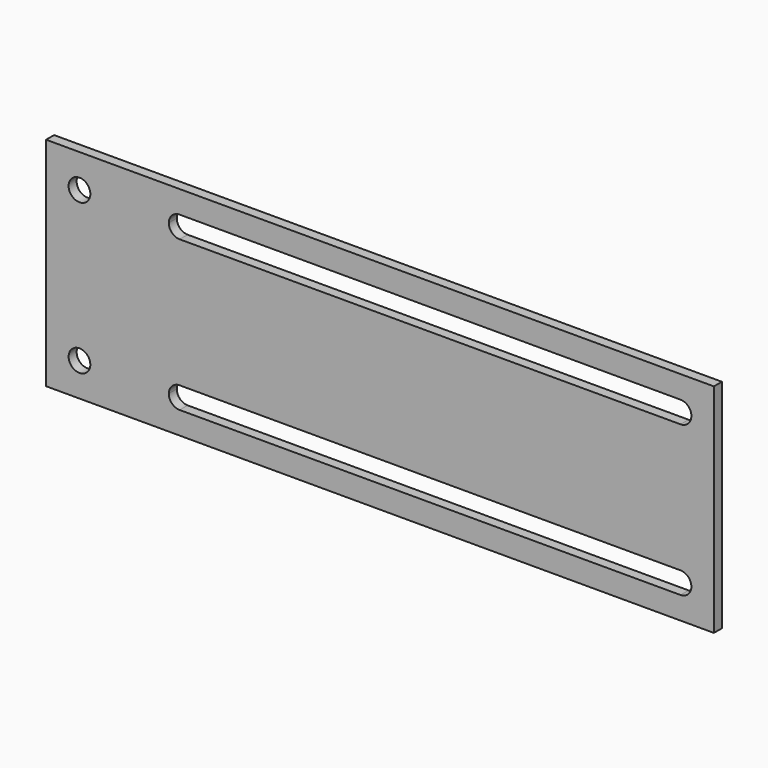
from build123d import *

# Parameters (mm, degrees)
F1_DEPTH = 3


# Not quite as in the source:
# - a feature names something its author has since deleted; it is built from what else it names


with BuildPart() as f1:
    # F0 (on Front) → F1 (new body)
    with BuildSketch(Plane.XZ):
        with BuildLine():
            Line((0, 65), (0, 55))
            Line((0, 55), (6.75, 55))
            ThreePointArc((6.75, 55), (10, 58.25), (13.25, 55))
            Line((13.25, 55), (36.75, 55))
            ThreePointArc((36.75, 55), (37.7019029611, 57.2980970389), (40, 58.25))
            Line((40, 58.25), (100, 58.25))
            Line((100, 58.25), (100, 65))
            Line((100, 65), (0, 65))
        make_face()
        with BuildLine():
            Line((0, 55), (0, 32.5))
            Line((0, 32.5), (30, 32.5))
            Line((30, 32.5), (100, 32.5))
            Line((100, 32.5), (100, 51.75))
            Line((100, 51.75), (40, 51.75))
            ThreePointArc((40, 51.75), (37.7019029611, 52.7019029611), (36.75, 55))
            Line((36.75, 55), (13.25, 55))
            ThreePointArc((13.25, 55), (10, 51.75), (6.75, 55))
            Line((6.75, 55), (0, 55))
        make_face()
        with BuildLine():
            Line((0, 32.5), (0, 10))
            Line((0, 10), (6.75, 10))
            ThreePointArc((6.75, 10), (10, 13.25), (13.25, 10))
            Line((13.25, 10), (30, 10))
            Line((30, 10), (30, 32.5))
            Line((30, 32.5), (0, 32.5))
        make_face()
        with BuildLine():
            Line((0, 10), (0, 0))
            Line((0, 0), (30, 0))
            Line((30, 0), (30, 10))
            Line((30, 10), (13.25, 10))
            ThreePointArc((13.25, 10), (10, 6.75), (6.75, 10))
            Line((6.75, 10), (0, 10))
        make_face()
        with BuildLine():
            Line((30, 32.5), (30, 10))
            Line((30, 10), (36.75, 10))
            ThreePointArc((36.75, 10), (37.7019029611, 12.2980970389), (40, 13.25))
            Line((40, 13.25), (100, 13.25))
            Line((100, 13.25), (100, 32.5))
            Line((100, 32.5), (30, 32.5))
        make_face()
        with BuildLine():
            Line((30, 10), (30, 0))
            Line((30, 0), (100, 0))
            Line((100, 0), (100, 6.75))
            Line((100, 6.75), (40, 6.75))
            ThreePointArc((40, 6.75), (37.7019029611, 7.7019029611), (36.75, 10))
            Line((36.75, 10), (30, 10))
        make_face()
        with BuildLine():
            Line((100, 32.5), (200, 32.5))
            Line((200, 32.5), (200, 65))
            Line((200, 65), (100, 65))
            Line((100, 65), (100, 58.25))
            Line((100, 58.25), (190, 58.25))
            ThreePointArc((190, 58.25), (192.2980970389, 57.2980970389), (193.25, 55))
            ThreePointArc((193.25, 55), (192.2980970389, 52.7019029611), (190, 51.75))
            Line((190, 51.75), (100, 51.75))
            Line((100, 51.75), (100, 32.5))
        make_face()
        with BuildLine():
            Line((100, 6.75), (100, 0))
            Line((100, 0), (200, 0))
            Line((200, 0), (200, 32.5))
            Line((200, 32.5), (100, 32.5))
            Line((100, 32.5), (100, 13.25))
            Line((100, 13.25), (190, 13.25))
            ThreePointArc((190, 13.25), (192.2980970389, 12.2980970389), (193.25, 10))
            ThreePointArc((193.25, 10), (192.2980970389, 7.7019029611), (190, 6.75))
            Line((190, 6.75), (100, 6.75))
        make_face()
    extrude(amount=F1_DEPTH)


solid = f1.part
